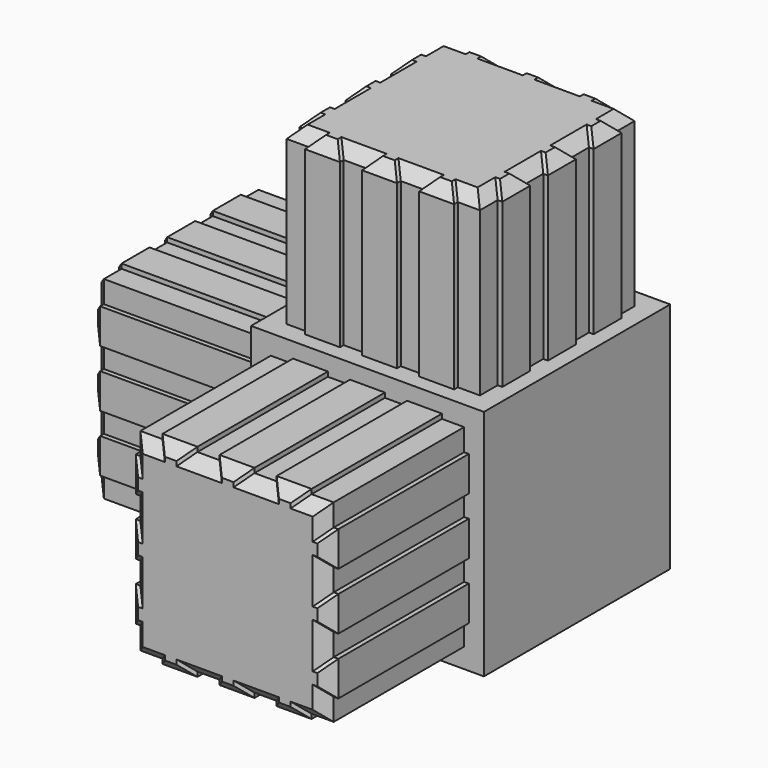
from build123d import *

# Parameters (mm, degrees)
F0_W     = 20
F0_H     = 20
F1_DEPTH = 20
F2_DEPTH = 15
F3_SIZE  = 1
F4_ANGLE = 90
F6_ANGLE = 90


with BuildPart() as f1:
    # F0 (on Top) → F1 (new body)
    with BuildSketch(Plane.XY):
        Rectangle(F0_W, F0_H)
        Polygon((-8.3, 6.4), (-8.3, 8.3), (-6.4, 8.3), (-6.4, 8.7), (-3.4, 8.7), (-3.4, 8.3), (-1.5, 8.3), (-1.5, 8.7), (1.5, 8.7), (1.5, 8.3), (3.4, 8.3), (3.4, 8.7), (6.4, 8.7), (6.4, 8.3), (8.3, 8.3), (8.3, 6.4), (8.7, 6.4), (8.7, 3.4), (8.3, 3.4), (8.3, 1.5), (8.7, 1.5), (8.7, -1.5), (8.3, -1.5), (8.3, -3.4), (8.7, -3.4), (8.7, -6.4), (8.3, -6.4), (8.3, -8.3), (6.4, -8.3), (6.4, -8.7), (3.4, -8.7), (3.4, -8.3), (1.5, -8.3), (1.5, -8.7), (-1.5, -8.7), (-1.5, -8.3), (-3.4, -8.3), (-3.4, -8.7), (-6.4, -8.7), (-6.4, -8.3), (-8.3, -8.3), (-8.3, -6.4), (-8.7, -6.4), (-8.7, -3.4), (-8.3, -3.4), (-8.3, -1.5), (-8.7, -1.5), (-8.7, 1.5), (-8.3, 1.5), (-8.3, 3.4), (-8.7, 3.4), (-8.7, 6.4), align=None, mode=Mode.SUBTRACT)
        Polygon((-6.4, 8.3), (-8.3, 8.3), (-8.3, 6.4), (-8.7, 6.4), (-8.7, 3.4), (-8.3, 3.4), (-8.3, 1.5), (-8.7, 1.5), (-8.7, -1.5), (-8.3, -1.5), (-8.3, -3.4), (-8.7, -3.4), (-8.7, -6.4), (-8.3, -6.4), (-8.3, -8.3), (-6.4, -8.3), (-6.4, -8.7), (-3.4, -8.7), (-3.4, -8.3), (-1.5, -8.3), (-1.5, -8.7), (1.5, -8.7), (1.5, -8.3), (3.4, -8.3), (3.4, -8.7), (6.4, -8.7), (6.4, -8.3), (8.3, -8.3), (8.3, -6.4), (8.7, -6.4), (8.7, -3.4), (8.3, -3.4), (8.3, -1.5), (8.7, -1.5), (8.7, 1.5), (8.3, 1.5), (8.3, 3.4), (8.7, 3.4), (8.7, 6.4), (8.3, 6.4), (8.3, 8.3), (6.4, 8.3), (6.4, 8.7), (3.4, 8.7), (3.4, 8.3), (1.5, 8.3), (1.5, 8.7), (-1.5, 8.7), (-1.5, 8.3), (-3.4, 8.3), (-3.4, 8.7), (-6.4, 8.7), align=None)
    extrude(amount=-F1_DEPTH)


with BuildPart() as f2:
    # F0 (on Top) → F2 (new body)
    with BuildSketch(Plane.XY):
        Polygon((-6.4, 8.3), (-8.3, 8.3), (-8.3, 6.4), (-8.7, 6.4), (-8.7, 3.4), (-8.3, 3.4), (-8.3, 1.5), (-8.7, 1.5), (-8.7, -1.5), (-8.3, -1.5), (-8.3, -3.4), (-8.7, -3.4), (-8.7, -6.4), (-8.3, -6.4), (-8.3, -8.3), (-6.4, -8.3), (-6.4, -8.7), (-3.4, -8.7), (-3.4, -8.3), (-1.5, -8.3), (-1.5, -8.7), (1.5, -8.7), (1.5, -8.3), (3.4, -8.3), (3.4, -8.7), (6.4, -8.7), (6.4, -8.3), (8.3, -8.3), (8.3, -6.4), (8.7, -6.4), (8.7, -3.4), (8.3, -3.4), (8.3, -1.5), (8.7, -1.5), (8.7, 1.5), (8.3, 1.5), (8.3, 3.4), (8.7, 3.4), (8.7, 6.4), (8.3, 6.4), (8.3, 8.3), (6.4, 8.3), (6.4, 8.7), (3.4, 8.7), (3.4, 8.3), (1.5, 8.3), (1.5, 8.7), (-1.5, 8.7), (-1.5, 8.3), (-3.4, 8.3), (-3.4, 8.7), (-6.4, 8.7), align=None)
    extrude(amount=F2_DEPTH)

    # F3
    f3_edges = [f2.edges().sort_by_distance(p)[0] for p in [
        (-7.35, 8.3, 15),
        (-8.3, 7.35, 15),
        (-8.5, 6.4, 15),
        (-8.7, 4.9, 15),
        (-8.5, 3.4, 15),
        (-8.3, 2.45, 15),
        (-8.5, 1.5, 15),
        (-8.7, 0, 15),
        (-8.5, -1.5, 15),
        (-8.3, -2.45, 15),
        (-8.5, -3.4, 15),
        (-8.7, -4.9, 15),
        (-8.5, -6.4, 15),
        (-8.3, -7.35, 15),
        (-7.35, -8.3, 15),
        (-6.4, -8.5, 15),
        (-4.9, -8.7, 15),
        (-3.4, -8.5, 15),
        (-2.45, -8.3, 15),
        (-1.5, -8.5, 15),
        (0, -8.7, 15),
        (1.5, -8.5, 15),
        (2.45, -8.3, 15),
        (3.4, -8.5, 15),
        (4.9, -8.7, 15),
        (6.4, -8.5, 15),
        (7.35, -8.3, 15),
        (8.3, -7.35, 15),
        (8.5, -6.4, 15),
        (8.7, -4.9, 15),
        (8.5, -3.4, 15),
        (8.3, -2.45, 15),
        (8.5, -1.5, 15),
        (8.7, 0, 15),
        (8.5, 1.5, 15),
        (8.3, 2.45, 15),
        (8.5, 3.4, 15),
        (8.7, 4.9, 15),
        (8.5, 6.4, 15),
        (8.3, 7.35, 15),
        (7.35, 8.3, 15),
        (6.4, 8.5, 15),
        (4.9, 8.7, 15),
        (3.4, 8.5, 15),
        (2.45, 8.3, 15),
        (1.5, 8.5, 15),
        (0, 8.7, 15),
        (-1.5, 8.5, 15),
        (-2.45, 8.3, 15),
        (-3.4, 8.5, 15),
        (-4.9, 8.7, 15),
        (-6.4, 8.5, 15),
    ]]
    chamfer(f3_edges, length=F3_SIZE)


with BuildPart() as f4_1:
    # F4: copy of F2
    add(f2.part.rotate(Axis((10, 0, 0), (0, -1, 0)), F4_ANGLE))


with BuildPart() as f4_1_1:
    # F5: moved
    add(f4_1.part.moved(Location((-20, 0, 0))))


with BuildPart() as f6_1:
    # F6: copy of F4_1
    add(f4_1_1.part.rotate(Axis((-10, 10, -10), (0, 0, 1)), F6_ANGLE))


with BuildPart() as f6_1_1:
    # F7: moved
    add(f6_1.part.moved(Location((0, -20, 0))))


solid = Compound([f1.part, f2.part, f4_1_1.part, f6_1_1.part])
